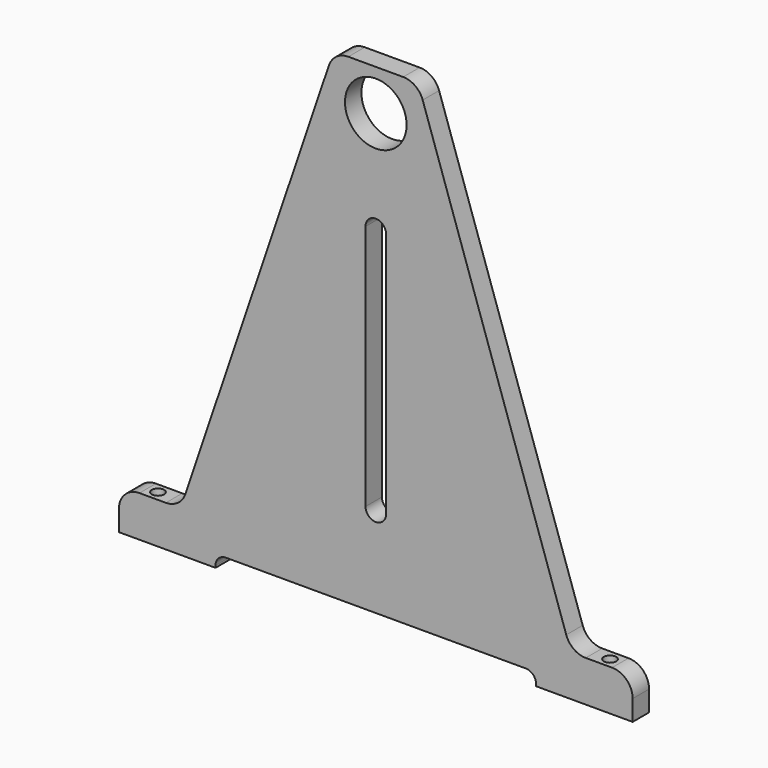
from build123d import *

# Parameters (mm, degrees)
F0_R     = 15
F1_DEPTH = 10
F3_D     = 6


# Not quite as in the source:
# - a feature names something its author has since deleted; it is built from what else it names


with BuildPart() as f1:
    # F0 (on Front) → F1 (new body)
    with BuildSketch(Plane.XZ):
        with BuildLine():
            Line((-125, -10), (-125, -20))
            Line((-125, -20), (-78, -20))
            Line((-78, -20), (-78, -19))
            ThreePointArc((-78, -19), (-76.5355339059, -15.4644660941), (-73, -14))
            Line((-73, -14), (73, -14))
            ThreePointArc((73, -14), (76.5355339059, -15.4644660941), (78, -19))
            Line((78, -19), (78, -20))
            Line((78, -20), (125, -20))
            Line((125, -20), (125, -10))
            ThreePointArc((125, -10), (122.0710678119, -2.9289321881), (115, 0))
            Line((115, 0), (102.1720946881, 0))
            ThreePointArc((102.1720946881, 0), (96.3439915213, 1.8739177043), (92.7001654958, 6.7933573047))
            Line((92.7001654958, 6.7933573047), (22.8206678375, 213.2066426953))
            ThreePointArc((22.8206678375, 213.2066426953), (19.176841812, 218.1260822957), (13.3487386452, 220))
            Line((13.3487386452, 220), (0, 220))
            Line((0, 220), (-13.3487386452, 220))
            ThreePointArc((-13.3487386452, 220), (-19.176841812, 218.1260822957), (-22.8206678375, 213.2066426953))
            Line((-22.8206678375, 213.2066426953), (-92.7001654958, 6.7933573047))
            ThreePointArc((-92.7001654958, 6.7933573047), (-96.3439915213, 1.8739177043), (-102.1720946881, 0))
            Line((-102.1720946881, 0), (-115, 0))
            ThreePointArc((-115, 0), (-122.0710678119, -2.9289321881), (-125, -10))
        make_face()
        with BuildLine():
            ThreePointArc((5, 30), (0, 25), (-5, 30))
            Line((-5, 30), (-5, 150))
            ThreePointArc((-5, 150), (0, 155), (5, 150))
            Line((5, 150), (5, 30))
        make_face(mode=Mode.SUBTRACT)
        with Locations((0, 200)):
            Circle(F0_R, mode=Mode.SUBTRACT)
    extrude(amount=F1_DEPTH)

    # F3 (through all)
    with Locations(Plane.XY):
        with Locations((-110, -5), (110, -5)):
            Hole(F3_D / 2)


solid = f1.part
